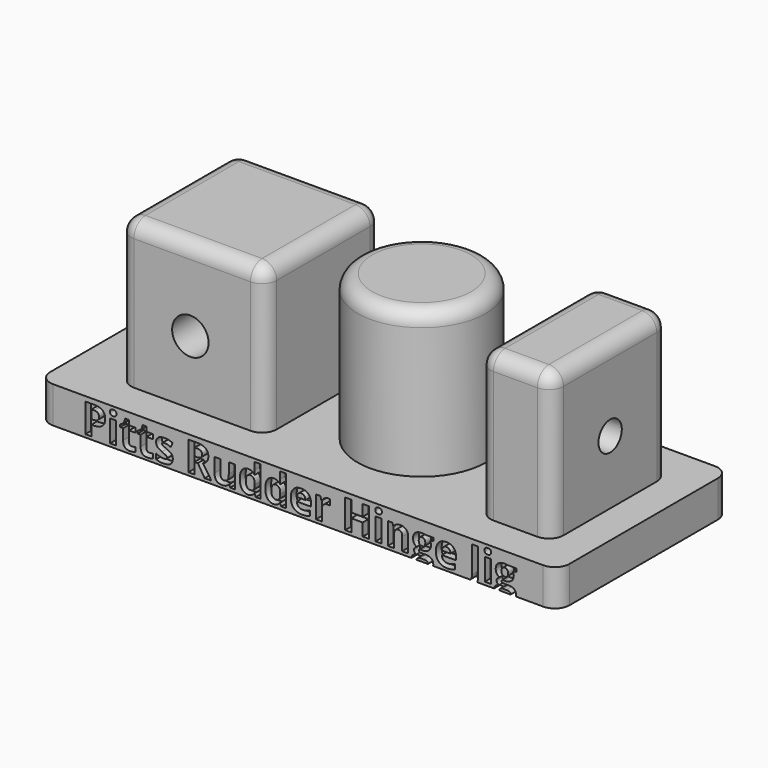
from build123d import *

# Parameters (mm, degrees)
F0_R         = 11.176
F1_DEPTH     = 25.4
F0_W         = 25.4
F0_H         = 25.4
F0_W_2       = 12.7
F2_R         = 3.175
F3_DEPTH     = 25.4
F4_R         = 2.54
F5_DEPTH     = 15.24
F6_W         = 90.5163660645
F6_H         = 37.4072734267
F7_DEPTH     = 6.35
F8_R         = 2.54
F8_2_R       = 2.54
F8_3_R       = 2.54
F8_4_R       = 2.54
F9_TEXT_SIZE = 7.027393115
F10_DEPTH    = 1.27


# Not quite as in the source:
# - Text() gives the source's letters only with a copy of the font that has no kerning and outlines rounded to 1/6400 em; it was checked with that copy


with BuildPart() as f1:
    # F0 (on Top) → F1 (new body)
    with BuildSketch(Plane.XY):
        Circle(F0_R)
    extrude(amount=F1_DEPTH)

    # F8#4
    f8_4_edges = [f1.edges().sort_by_distance(p)[0] for p in [
        (-11.176, 0, 25.4),
    ]]
    fillet(f8_4_edges, radius=F8_4_R)


with BuildPart() as f1b:
    # F0 (on Top) → F1, piece 2 (new body)
    with BuildSketch(Plane.XY):
        with Locations((-29.8450030386, 0)):
            Rectangle(F0_W, F0_H)
    extrude(amount=F1_DEPTH)

    # F2 (on Front) → F3 (cut, symmetric)
    with BuildSketch(Plane.XZ):
        with Locations((-30.1625, 11.1125)):
            Circle(F2_R)
    extrude(amount=F3_DEPTH, both=True, mode=Mode.SUBTRACT)

    # F8#2
    f8_2_edges = [f1b.edges().sort_by_distance(p)[0] for p in [
        (-17.145003, 12.7, 12.7),
        (-42.545003, 12.7, 12.7),
        (-42.545003, -12.7, 12.7),
        (-17.145003, -12.7, 12.7),
        (-29.845003, 12.7, 25.4),
        (-17.145003, 0, 25.4),
        (-29.845003, -12.7, 25.4),
        (-42.545003, 0, 25.4),
    ]]
    fillet(f8_2_edges, radius=F8_2_R)


with BuildPart() as f1c:
    # F0 (on Top) → F1, piece 3 (new body)
    with BuildSketch(Plane.XY):
        with Locations((26.4968145639, 0)):
            Rectangle(F0_W_2, F0_H)
    extrude(amount=F1_DEPTH)

    # F4 (on face) → F5 (cut)
    with BuildSketch(Plane.YZ.offset(32.8468145639)):
        with Locations((0, 11.1125)):
            Circle(F4_R)
    extrude(amount=-F5_DEPTH, mode=Mode.SUBTRACT)

    # F8
    f8_edges = [f1c.edges().sort_by_distance(p)[0] for p in [
        (20.146815, 12.7, 12.7),
        (32.846815, 12.7, 12.7),
        (20.146815, -12.7, 12.7),
        (32.846815, -12.7, 12.7),
        (26.496815, -12.7, 25.4),
        (26.496815, 12.7, 25.4),
        (20.146815, 0, 25.4),
        (32.846815, 0, 25.4),
    ]]
    fillet(f8_edges, radius=F8_R)


with BuildPart() as f7:
    # F6 (on Top) → F7 (new body)
    with BuildSketch(Plane.XY):
        with Locations((-6.5231844783, -0.0577261671)):
            Rectangle(F6_W, F6_H)
    extrude(amount=-F7_DEPTH)

    # F8#3
    f8_3_edges = [f7.edges().sort_by_distance(p)[0] for p in [
        (-51.781368, -18.761363, -3.175),
        (-51.781368, 18.645911, -3.175),
        (38.734999, -18.761363, -3.175),
        (38.734999, 18.645911, -3.175),
    ]]
    fillet(f8_3_edges, radius=F8_3_R)

    # F9 (on face) → F10 (cut)
    with BuildSketch(Plane.XZ.offset(18.7613628805)):
        with Locations((-44.2523558146, -5.8386084639)):
            Text('Pitts Rudder Hinge Jig', F9_TEXT_SIZE, font='Open Sans', font_style=FontStyle.BOLD, text_align=(TextAlign.LEFT, TextAlign.BOTTOM))
    extrude(amount=-F10_DEPTH, mode=Mode.SUBTRACT)


solid = Compound([f1.part, f1b.part, f1c.part, f7.part])
